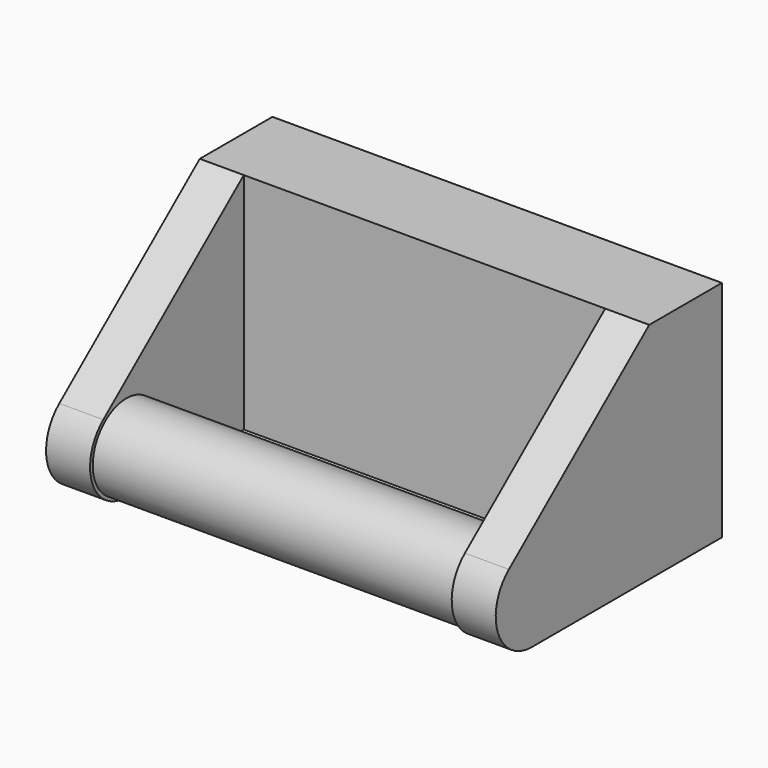
from build123d import *

# Parameters (mm, degrees)
F0_W      = 15.83
F0_H      = 7.89
F1_DEPTH  = 3.2
F3_DEPTH  = 1.55
F4_R      = 1.59
F6_DEPTH  = 1.55
F7_R      = 1.59
F8_DEPTH  = 1.55
F9_R      = 1.48
F10_DEPTH = 12.83
F11_T     = -1.57
F12_R     = 1.535
F12_R_2   = 0.765
F13_DEPTH = 1.6


with BuildPart() as f1:
    # F0 (on Front) → F1 (new body)
    with BuildSketch(Plane.XZ):
        with Locations((-28.0223558657, 18.9167669917)):
            Rectangle(F0_W, F0_H)
    extrude(amount=F1_DEPTH)

    # F2 (on face) → F3 (join)
    with BuildSketch(Plane.YZ.offset(-20.1073558657)):
        Polygon((-12.81, 14.9717669917), (-3.2, 14.9717669917), (-3.2, 22.8617669917), align=None)
    extrude(amount=-F3_DEPTH)

    # F4
    f4_edges = [f1.edges().sort_by_distance(p)[0] for p in [
        (-20.882356, -12.81, 14.971767),
    ]]
    fillet(f4_edges, radius=F4_R)

    # F5 (on face) → F6 (join)
    with BuildSketch(Plane(origin=(-35.9373558657, 0, 0), x_dir=(0, -1, 0), z_dir=(-1, 0, 0))):
        Polygon((3.2, 22.8617669917), (3.2, 14.9717669917), (12.8218363971, 14.9717669917), align=None)
    extrude(amount=-F6_DEPTH)

    # F7
    f7_edges = [f1.edges().sort_by_distance(p)[0] for p in [
        (-35.162356, -12.821836, 14.971767),
    ]]
    fillet(f7_edges, radius=F7_R)


with BuildPart() as f8:
    # F8 (new): a face of the model
    f8_faces = [f1.part.faces().sort_by_distance(p)[0] for p in [
        (-35.9373558657, -4.069759588, 18.2879557139),
    ]]
    extrude(f8_faces, amount=-F8_DEPTH)


with BuildPart() as f1_1:
    add(f1.part)

    add(f8.part)  # F10 merges F8
    # F9 (on face) → F10 (join)
    with BuildSketch(Plane(origin=(-21.6573558657, 0, 0), x_dir=(0, -1, 0), z_dir=(-1, 0, 0))):
        with Locations((8.367674268, 16.5617669917)):
            Circle(F9_R)
    extrude(amount=F10_DEPTH)

    # F11
    f11_openings = [f1_1.faces().sort_by_distance(p)[0] for p in [
        (-28.022356, 0, 18.916767),
    ]]
    offset(amount=F11_T, openings=f11_openings)

    # F12 (on face) → F13 (join)
    with BuildSketch(Plane(origin=(0, -1.63, 0), x_dir=(-1, 0, 0), z_dir=(0, 1, 0))):
        with Locations((28.0223558657, 18.9167669917)):
            Circle(F12_R)
        with Locations((28.0223558657, 18.9167669917)):
            Circle(F12_R_2, mode=Mode.SUBTRACT)
    extrude(amount=F13_DEPTH)


solid = f1_1.part
